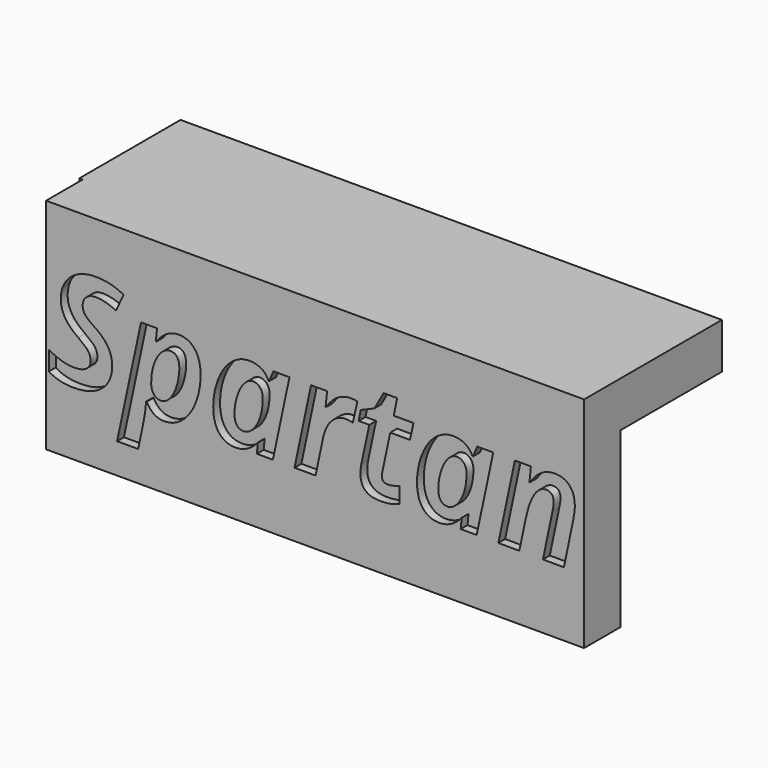
from build123d import *

# Parameters (mm, degrees)
F0_W         = 94.2432358861
F0_H         = 38.35272789
F1_DEPTH     = 8
F2_W         = 94.8291271925
F2_H         = 22.1755299717
F3_DEPTH     = 8
F4_TEXT_SIZE = 25.0469959583
F5_DEPTH     = 1.5


# Not quite as in the source:
# - Text() gives the source's letters only with a copy of the font that has no kerning and outlines rounded to 1/6400 em; it was checked with that copy


with BuildPart() as f1:
    # F0 (on Front) → F1 (new body)
    with BuildSketch(Plane.XZ):
        with Locations((-47.121617943, -19.176363945)):
            Rectangle(F0_W, F0_H)
    extrude(amount=F1_DEPTH)

    # F2 (on Top) → F3 (join)
    with BuildSketch(Plane.XY):
        with Locations((-47.4145635962, 11.0877649859)):
            Rectangle(F2_W, F2_H)
    extrude(amount=-F3_DEPTH)

    # F4 (on face) → F5 (cut)
    with BuildSketch(Plane.XZ.offset(8)):
        with Locations((-94.2432358861, -27.029673299)):
            Text('Spartan', F4_TEXT_SIZE, font='Open Sans', font_style=FontStyle.BOLDITALIC, text_align=(TextAlign.LEFT, TextAlign.BOTTOM))
    extrude(amount=-F5_DEPTH, mode=Mode.SUBTRACT)


solid = f1.part
